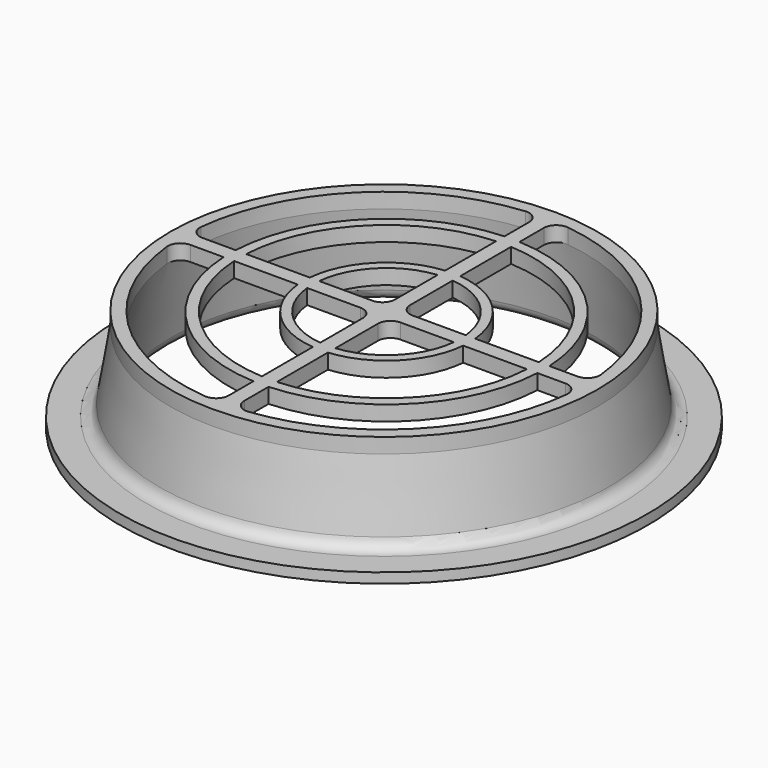
from build123d import *

# Parameters (mm, degrees)
F1_FACE_R   = 17
F1_FACE_R_2 = 16
F3_DEPTH    = 1.2
F4_T1_DEPTH = 1.2


# Not quite as in the source:
# - a fillet or chamfer that OpenCascade refuses, or shapes differently, is made with other operations: its cross-section is extruded or revolved along the edge and cut away or added


with BuildPart() as f1:
    # F0 (on Front) → F1 (revolve)
    with BuildSketch(Plane.XZ):
        with BuildLine():
            Line((-5, -6.2), (-5, -7))
            Line((-5, -7), (-1.8672954017, -7))
            ThreePointArc((-1.8672954017, -7), (-1.2120936603, -6.755453955), (-0.877345908, -6.1414213562))
            Line((-0.877345908, -6.1414213562), (0, 0))
            Line((0, 0), (-1, 0))
            Line((-1, 0), (-1.8643923288, -5.3592324388))
            ThreePointArc((-1.8643923288, -5.3592324388), (-2.2032633542, -5.9613253046), (-2.8516334496, -6.2))
            Line((-2.8516334496, -6.2), (-5, -6.2))
        make_face()
    revolve(axis=Axis((16, 0, -3.4995676855), (0, 0, -1)))

    # F1_face (on face) + F2 (on Top) → F3 (join)
    with BuildSketch(Plane(origin=(16, 0, 0), x_dir=(1, 0, 0), z_dir=(0, 0, 1))):
        Circle(F1_FACE_R)
        Circle(F1_FACE_R_2, mode=Mode.SUBTRACT)
    with BuildSketch(Plane.XY):
        with BuildLine():
            Line((3.7233340059, 0.6), (0.0112539579, 0.6))
            ThreePointArc((0.0112539579, 0.6), (0, 0), (0.0112539579, -0.6))
            Line((0.0112539579, -0.6), (3.7233340059, -0.6))
            ThreePointArc((3.7233340059, -0.6), (7.3688969309, -8.8359634953), (15.6048604261, -12.4815264202))
            Line((15.6048604261, -12.4815264202), (15.6048604261, -15.9951200282))
            ThreePointArc((15.6048604261, -15.9951200282), (16.2050046444, -15.9986866053), (16.8048604261, -15.9797434177))
            Line((16.8048604261, -15.9797434177), (16.8048604261, -12.4815264202))
            ThreePointArc((16.8048604261, -12.4815264202), (25.0408239214, -8.8359634953), (28.6863868464, -0.6))
            Line((28.6863868464, -0.6), (31.9887460421, -0.6))
            ThreePointArc((31.9887460421, -0.6), (31.9971862631, -0.3000527668), (32, 0))
            ThreePointArc((32, 0), (31.9971862631, 0.3000527668), (31.9887460421, 0.6))
            Line((31.9887460421, 0.6), (28.6863868464, 0.6))
            ThreePointArc((28.6863868464, 0.6), (25.0408239214, 8.8359634953), (16.8048604261, 12.4815264202))
            Line((16.8048604261, 12.4815264202), (16.8048604261, 15.9797434177))
            ThreePointArc((16.8048604261, 15.9797434177), (16.2050046444, 15.9986866053), (15.6048604261, 15.9951200282))
            Line((15.6048604261, 15.9951200282), (15.6048604261, 12.4815264202))
            ThreePointArc((15.6048604261, 12.4815264202), (7.3688969309, 8.8359634953), (3.7233340059, 0.6))
        make_face()
        with BuildLine():
            ThreePointArc((15.6048604261, -11.6414250608), (7.9622037717, -8.2426566544), (4.5634353654, -0.6))
            Line((4.5634353654, -0.6), (9.6268322864, -0.6))
            ThreePointArc((9.6268322864, -0.6), (11.5341830552, -4.6706773709), (15.6048604261, -6.5780281397))
            Line((15.6048604261, -6.5780281397), (15.6048604261, -11.6414250608))
        make_face(mode=Mode.SUBTRACT)
        with BuildLine():
            ThreePointArc((15.6048604261, -5.8326828273), (12.0587665437, -4.1460938824), (10.3721775989, -0.6))
            Line((10.3721775989, -0.6), (14.6048604261, -0.6))
            ThreePointArc((14.6048604261, -0.6), (15.3119672073, -0.8928932188), (15.6048604261, -1.6))
            Line((15.6048604261, -1.6), (15.6048604261, -5.8326828273))
        make_face(mode=Mode.SUBTRACT)
        with BuildLine():
            ThreePointArc((16.8048604261, -6.5780281397), (20.875537797, -4.6706773709), (22.7828885658, -0.6))
            Line((22.7828885658, -0.6), (27.8462854869, -0.6))
            ThreePointArc((27.8462854869, -0.6), (24.4475170805, -8.2426566544), (16.8048604261, -11.6414250608))
            Line((16.8048604261, -11.6414250608), (16.8048604261, -6.5780281397))
        make_face(mode=Mode.SUBTRACT)
        with BuildLine():
            ThreePointArc((22.0375432534, -0.6), (20.3509543085, -4.1460938824), (16.8048604261, -5.8326828273))
            Line((16.8048604261, -5.8326828273), (16.8048604261, -1.6))
            ThreePointArc((16.8048604261, -1.6), (17.0977536449, -0.8928932188), (17.8048604261, -0.6))
            Line((17.8048604261, -0.6), (22.0375432534, -0.6))
        make_face(mode=Mode.SUBTRACT)
        with BuildLine():
            ThreePointArc((10.3721775989, 0.6), (12.0587665437, 4.1460938824), (15.6048604261, 5.8326828273))
            Line((15.6048604261, 5.8326828273), (15.6048604261, 1.6))
            ThreePointArc((15.6048604261, 1.6), (15.3119672073, 0.8928932188), (14.6048604261, 0.6))
            Line((14.6048604261, 0.6), (10.3721775989, 0.6))
        make_face(mode=Mode.SUBTRACT)
        with BuildLine():
            ThreePointArc((4.5634353654, 0.6), (7.9622037717, 8.2426566544), (15.6048604261, 11.6414250608))
            Line((15.6048604261, 11.6414250608), (15.6048604261, 6.5780281397))
            ThreePointArc((15.6048604261, 6.5780281397), (11.5341830552, 4.6706773709), (9.6268322864, 0.6))
            Line((9.6268322864, 0.6), (4.5634353654, 0.6))
        make_face(mode=Mode.SUBTRACT)
        with BuildLine():
            Line((16.8048604261, 1.6), (16.8048604261, 5.8326828273))
            ThreePointArc((16.8048604261, 5.8326828273), (20.3509543085, 4.1460938824), (22.0375432534, 0.6))
            Line((22.0375432534, 0.6), (17.8048604261, 0.6))
            ThreePointArc((17.8048604261, 0.6), (17.0977536449, 0.8928932188), (16.8048604261, 1.6))
        make_face(mode=Mode.SUBTRACT)
        with BuildLine():
            Line((16.8048604261, 6.5780281397), (16.8048604261, 11.6414250608))
            ThreePointArc((16.8048604261, 11.6414250608), (24.4475170805, 8.2426566544), (27.8462854869, 0.6))
            Line((27.8462854869, 0.6), (22.7828885658, 0.6))
            ThreePointArc((22.7828885658, 0.6), (20.875537797, 4.6706773709), (16.8048604261, 6.5780281397))
        make_face(mode=Mode.SUBTRACT)
    extrude(amount=F3_DEPTH)

    # F4: fillet of radius 1 on 8 edges, made by hand

    # F4_s2 → F4_t1 (join)
    with BuildSketch(Plane.XY):
        with BuildLine():
            ThreePointArc((14.5118511212, 15.9306438324), (15.2782810581, 15.6742381227), (15.6048604261, 14.9349785929))
            Line((15.6048604261, 14.9349785929), (15.6048604261, 15.9951200282))
            ThreePointArc((15.6048604261, 15.9951200282), (15.0578040841, 15.9722342475), (14.5118511212, 15.9306438324))
        make_face()
        with BuildLine():
            ThreePointArc((17.9251844545, 15.8837547455), (17.1416576021, 15.6394597938), (16.8048604261, 14.8910200739))
            Line((16.8048604261, 14.8910200739), (16.8048604261, 15.9797434177))
            ThreePointArc((16.8048604261, 15.9797434177), (17.3658659227, 15.9415937184), (17.9251844545, 15.8837547455))
        make_face()
        with BuildLine():
            ThreePointArc((31.9087173867, -1.7066666667), (31.6582863368, -0.9316687448), (30.91442255, -0.6))
            Line((30.91442255, -0.6), (31.9887460421, -0.6))
            ThreePointArc((31.9887460421, -0.6), (31.9583276403, -1.1540272632), (31.9087173867, -1.7066666667))
        make_face()
        with BuildLine():
            ThreePointArc((31.9087173867, 1.7066666667), (31.6582863368, 0.9316687448), (30.91442255, 0.6))
            Line((30.91442255, 0.6), (31.9887460421, 0.6))
            ThreePointArc((31.9887460421, 0.6), (31.9583276403, 1.1540272632), (31.9087173867, 1.7066666667))
        make_face()
        with BuildLine():
            ThreePointArc((14.5118511212, -15.9306438324), (15.2782810581, -15.6742381227), (15.6048604261, -14.9349785929))
            Line((15.6048604261, -14.9349785929), (15.6048604261, -15.9951200282))
            ThreePointArc((15.6048604261, -15.9951200282), (15.0578040841, -15.9722342475), (14.5118511212, -15.9306438324))
        make_face()
        with BuildLine():
            ThreePointArc((17.9251844545, -15.8837547455), (17.1416576021, -15.6394597938), (16.8048604261, -14.8910200739))
            Line((16.8048604261, -14.8910200739), (16.8048604261, -15.9797434177))
            ThreePointArc((16.8048604261, -15.9797434177), (17.3658659227, -15.9415937184), (17.9251844545, -15.8837547455))
        make_face()
        with BuildLine():
            ThreePointArc((0.0912826133, 1.7066666667), (0.3417136632, 0.9316687448), (1.08557745, 0.6))
            Line((1.08557745, 0.6), (0.0112539579, 0.6))
            ThreePointArc((0.0112539579, 0.6), (0.0416723597, 1.1540272632), (0.0912826133, 1.7066666667))
        make_face()
        with BuildLine():
            ThreePointArc((0.0912826133, -1.7066666667), (0.3417136632, -0.9316687448), (1.08557745, -0.6))
            Line((1.08557745, -0.6), (0.0112539579, -0.6))
            ThreePointArc((0.0112539579, -0.6), (0.0416723597, -1.1540272632), (0.0912826133, -1.7066666667))
        make_face()
    extrude(amount=F4_T1_DEPTH)


solid = f1.part
